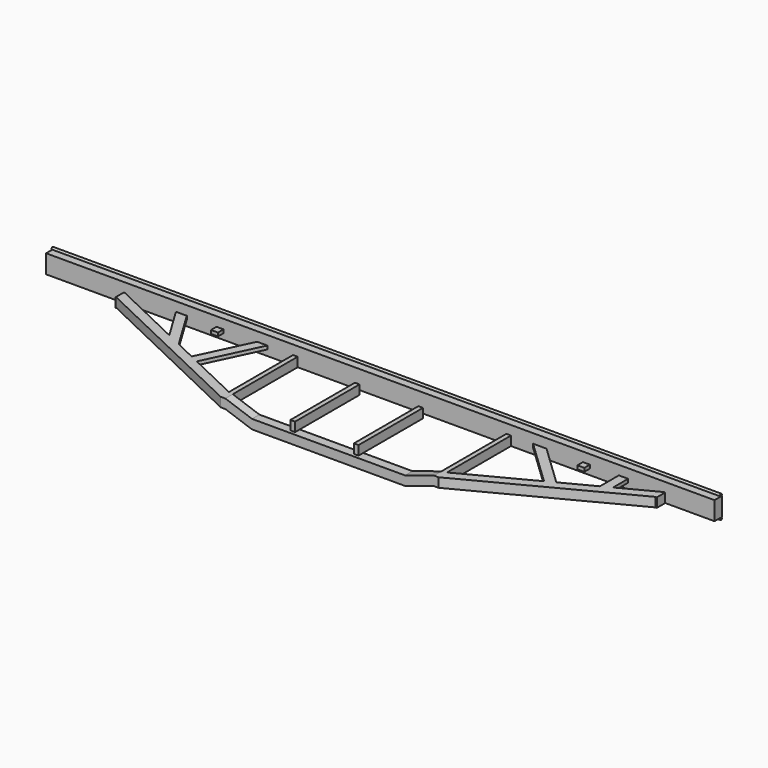
from build123d import *

# Parameters (mm, degrees)
F5_W      = 7321.55
F5_H      = 101.6
F6_DEPTH  = 203.2
F8_DEPTH  = 7321.55
F9_W      = 50.8
F9_H      = 990.6
F10_DEPTH = 101.6
F11_W     = 50.8
F11_H     = 882.65
F12_DEPTH = 101.6
F14_DEPTH = 101.6
F15_W     = 1676.4
F15_H     = 101.6
F16_DEPTH = 101.6
F17_W     = 76.2
F17_H     = 76.2
F18_DEPTH = 38.1


# Not quite as in the source:
# - a variable given as a bare number and used for a length is read in inches; the dataset says mm whatever the document's units were


with BuildPart() as f6:
    # F5 (on Top) → F6 (new body)
    with BuildSketch(Plane.XY):
        with Locations((0, -50.8)):
            Rectangle(F5_W, F5_H)
    extrude(amount=F6_DEPTH)

    # F7 (on face) → F8 (join)
    with BuildSketch(Plane.YZ.offset(3660.775)):
        with BuildLine():
            ThreePointArc((-9.5499023453, 203.596875), (-2.6676463326, 208.1127103629), (0, 215.9))
            ThreePointArc((0, 215.9), (-20.4872896371, 225.9323536674), (-15.8500976547, 203.596875))
            ThreePointArc((-15.8500976547, 203.596875), (-12.7, 206.375), (-9.5499023453, 203.596875))
        make_face()
        with BuildLine():
            ThreePointArc((-12.7, 203.2), (-14.2875, 203.2996093811), (-15.8500976547, 203.596875))
            ThreePointArc((-15.8500976547, 203.596875), (-15.8687682981, 203.3988277473), (-15.875, 203.2))
            Line((-15.875, 203.2), (-12.7, 203.2))
        make_face()
        with BuildLine():
            ThreePointArc((-9.525, 203.2), (-9.5312317019, 203.3988277473), (-9.5499023453, 203.596875))
            ThreePointArc((-9.5499023453, 203.596875), (-11.1125, 203.2996093811), (-12.7, 203.2))
            Line((-12.7, 203.2), (-9.525, 203.2))
        make_face()
        with BuildLine():
            Line((-9.525, 203.2), (-12.7, 203.2))
            Line((-12.7, 203.2), (-15.875, 203.2))
            ThreePointArc((-15.875, 203.2), (-12.7, 200.025), (-9.525, 203.2))
        make_face()
        with BuildLine():
            ThreePointArc((-9.5499023453, 203.596875), (-12.7, 206.375), (-15.8500976547, 203.596875))
            ThreePointArc((-15.8500976547, 203.596875), (-14.2875, 203.2996093811), (-12.7, 203.2))
            ThreePointArc((-12.7, 203.2), (-11.1125, 203.2996093811), (-9.5499023453, 203.596875))
        make_face()
        with BuildLine():
            ThreePointArc((-9.5499023453, -0.396875), (-12.7, -3.175), (-15.8500976547, -0.396875))
            ThreePointArc((-15.8500976547, -0.396875), (-20.4872896371, -22.7323536674), (0, -12.7))
            ThreePointArc((0, -12.7), (-2.6676463326, -4.9127103629), (-9.5499023453, -0.396875))
        make_face()
        with BuildLine():
            ThreePointArc((-12.7, 0), (-14.2875, -0.0996093811), (-15.8500976547, -0.396875))
            ThreePointArc((-15.8500976547, -0.396875), (-12.7, -3.175), (-9.5499023453, -0.396875))
            ThreePointArc((-9.5499023453, -0.396875), (-11.1125, -0.0996093811), (-12.7, 0))
        make_face()
        with BuildLine():
            Line((-12.7, 0), (-15.875, 0))
            ThreePointArc((-15.875, 0), (-15.8687682981, -0.1988277473), (-15.8500976547, -0.396875))
            ThreePointArc((-15.8500976547, -0.396875), (-14.2875, -0.0996093811), (-12.7, 0))
        make_face()
        with BuildLine():
            ThreePointArc((-9.5499023453, -0.396875), (-9.5312317019, -0.1988277473), (-9.525, 0))
            Line((-9.525, 0), (-12.7, 0))
            ThreePointArc((-12.7, 0), (-11.1125, -0.0996093811), (-9.5499023453, -0.396875))
        make_face()
    extrude(amount=-F8_DEPTH)

    # F9 (on Top) → F10 (join)
    with BuildSketch(Plane.XY):
        with Locations((-930.275, -596.9)):
            Rectangle(F9_W, F9_H)
        with Locations((1406.525, -596.9)):
            Rectangle(F9_W, F9_H)
    extrude(amount=F10_DEPTH)

    # F13 (on Top) → F14 (join)
    with BuildSketch(Plane.XY):
        Polygon((-955.675, -979.6417901101), (-2797.175, -101.6), (-2809.875, -101.6), (-2809.875, -214.1582098899), (-2797.175, -214.1582098899), (-955.675, -1092.2), align=None)
        Polygon((3108.325, -101.6), (1431.925, -977.565864756), (1431.925, -1092.2), (3108.325, -216.234135244), (3121.025, -216.234135244), (3121.025, -101.6), align=None)
    extrude(amount=F14_DEPTH)



with BuildPart() as f12:
    # F11 (on Top) → F12 (new body)
    with BuildSketch(Plane.XY):
        with Locations((-196.85, -612.775)):
            Rectangle(F11_W, F11_H)
    extrude(amount=F12_DEPTH)


with BuildPart() as f12b:
    # F11 (on Top) → F12, piece 2 (new body)
    with BuildSketch(Plane.XY):
        with Locations((498.475, -612.775)):
            Rectangle(F11_W, F11_H)
    extrude(amount=F12_DEPTH)


with BuildPart() as f6_1:
    add(f6.part)

    add(f12.part)  # F16 merges F12

    add(f12b.part)  # F16 merges F12b
    # F15 (on face) → F16 (join)
    with BuildSketch(Plane.XZ.offset(1092.2)):
        Polygon((-612.775, -101.6), (-612.775, 0), (-904.875, 101.6), (-904.875, 0), align=None)
        with Locations((225.425, -50.8)):
            Rectangle(F15_W, F15_H)
        Polygon((1381.125, 101.6), (1063.625, 0), (1063.625, -101.6), (1381.125, 0), align=None)
    extrude(amount=-F16_DEPTH)

    # F17 (on face) → F18 (join)
    with BuildSketch(Plane.XY.offset(101.6)):
        Polygon((-2119.6147810739, -101.6), (-2238.375, -101.6), (-2011.695225595, -476.1229797523), (-1844.759380981, -555.7193130884), align=None)
        with Locations((-1755.775, -139.5431798935)):
            Rectangle(F17_W, F17_H)
        Polygon((-1349.375, -101.6), (-1616.686877804, -664.4660896099), (-1524.9781313366, -708.1935465292), (-1236.8995581561, -101.6), align=None)
        Polygon((2276.3318432651, -536.339683256), (1820.4451820405, -101.6), (1673.225, -101.6), (2181.225, -586.0356676302), align=None)
        with Locations((2257.425, -139.7)):
            Rectangle(F17_W, F17_H)
        Polygon((2714.625, -101.6), (2613.025, -101.6), (2613.025, -360.4080964052), (2714.625, -307.3192561169), align=None)
    extrude(amount=-F18_DEPTH)


solid = f6_1.part
